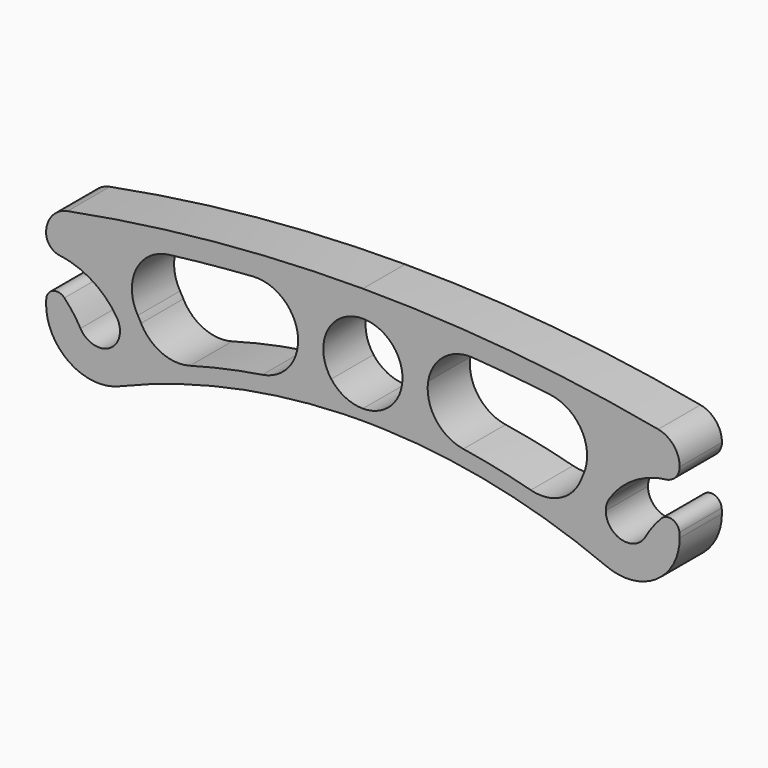
from build123d import *
from build123d import SkipClean  # not in build123d's __all__

# Parameters (mm, degrees)
F1_DEPTH    = 10
F3_R        = 5
F4_R        = 3
F5_R        = 2
F7_DEPTH    = 10.0010001
F8_T1_DEPTH = 10


# Not quite as in the source:
# - a fillet or chamfer that OpenCascade refuses, or shapes differently, is made with other operations: its cross-section is extruded or revolved along the edge and cut away or added


with BuildPart() as f1:
    # F0 (on Front) → F1 (new body)
    with BuildSketch(Plane.XZ):
        with BuildLine():
            ThreePointArc((-60, 9), (-57.6213157363, 8.9328971517), (-55.2831757887, 8.4904683961))
            ThreePointArc((-55.2831757887, 8.4904683961), (-45.1436514688, 8.7416176388), (-40, 0))
            ThreePointArc((-40, 0), (-41.6794970566, -5.5470019623), (-46.1538461538, -9.2307692308))
            ThreePointArc((-46.1538461538, -9.2307692308), (-25.4921003461, -2.7389543798), (-4, -0.0666851955))
            ThreePointArc((-4, -0.0666851955), (-4.6347028183, 2.6231856146), (-5.9814434357, 5.03659448))
            ThreePointArc((-5.9814434357, 5.03659448), (-6.715086481, 12.9015322824), (0, 17.061230866))
            Line((0, 17.061230866), (0, 22.061230866))
            ThreePointArc((0, 22.061230866), (-30.1526886016, 20.5420767676), (-60, 16))
            Line((-60, 16), (-60, 9))
        make_face()
        with BuildLine():
            ThreePointArc((-46.6427971379, 2.1746698468), (-46.1640639051, 1.1338404984), (-46, 0))
            ThreePointArc((-46, 0), (-48.9877288652, -3.8697941999), (-53.4876535749, -1.958640483))
            ThreePointArc((-53.4876535749, -1.958640483), (-55.921777017, 1.4722128283), (-59.0196729824, 4.3180434563))
            ThreePointArc((-59.0196729824, 4.3180434563), (-59.7518390528, 2.21396366), (-60, 0))
            ThreePointArc((-60, 0), (-55.5470019623, -8.3205029434), (-46.1538461538, -9.2307692308))
            ThreePointArc((-46.1538461538, -9.2307692308), (-41.6794970566, -5.5470019623), (-40, 0))
            ThreePointArc((-40, 0), (-45.1436514688, 8.7416176388), (-55.2831757887, 8.4904683961))
            ThreePointArc((-55.2831757887, 8.4904683961), (-50.3805281419, 6.1294058803), (-46.6427971379, 2.1746698468))
        make_face()
        with BuildLine():
            ThreePointArc((-5.9814434357, 5.03659448), (-4.6347028183, 2.6231856146), (-4, -0.0666851955))
            ThreePointArc((-4, -0.0666851955), (-2.0002779129, -0.0166724571), (0, 0))
            Line((0, 0), (0, 2.061230866))
            ThreePointArc((0, 2.061230866), (-3.3403014164, 2.846144385), (-5.9814434357, 5.03659448))
        make_face()
    extrude(amount=F1_DEPTH)

    # F2: F1 across plane


with BuildPart() as f1_1:
    add(f1.part, clean=False)
    with SkipClean():  # cleaning this boolean's faces spoils the solid; the shape is the same uncleaned
        add(f1.part.mirror(Plane.YZ), clean=False)

    # F3
    f3_edges = [f1_1.edges().sort_by_distance(p)[0] for p in [
        (-60, -5, 16),
        (60, -5, 16),
    ]]
    fillet(f3_edges, radius=F3_R)

    # F4
    f4_edges = [f1_1.edges().sort_by_distance(p)[0] for p in [
        (-60, -5, 9),
        (60, -5, 9),
    ]]
    fillet(f4_edges, radius=F4_R)

    # F5
    f5_edges = [f1_1.edges().sort_by_distance(p)[0] for p in [
        (-59.019673, -5, 4.318043),
        (59.019673, -5, 4.318043),
    ]]
    fillet(f5_edges, radius=F5_R)

    # F6 (on face) → F7 (cut, through all)
    with BuildSketch(Plane.XZ.offset(10)):
        with BuildLine():
            ThreePointArc((-7.8234196702, 2.7509433962), (-12.1811976175, 9.6949287705), (-11.2993718648, 17.8454836508))
            ThreePointArc((-11.2993718648, 17.8454836508), (-33.2415394106, 16.1887543276), (-55, 12.9065505808))
            ThreePointArc((-55, 12.9065505808), (-44.9636385736, 6.903343626), (-40, -3.685770432))
            ThreePointArc((-40, -3.685770432), (-24.1273224471, 0.6104154355), (-7.8234196702, 2.7509433962))
        make_face()
        with BuildLine():
            ThreePointArc((40, -3.685770432), (42.6359894717, 6.412330531), (50, 13.8076961402))
            ThreePointArc((50, 13.8076961402), (30.7161061945, 16.4632023612), (11.2993718648, 17.8454836508))
            ThreePointArc((11.2993718648, 17.8454836508), (12.1961499726, 15.2393294517), (12.5, 12.5))
            ThreePointArc((12.5, 12.5), (11.2703759005, 7.0936493768), (7.8234196702, 2.7509433962))
            ThreePointArc((7.8234196702, 2.7509433962), (24.1273224471, 0.6104154355), (40, -3.685770432))
        make_face()
    extrude(amount=-F7_DEPTH, mode=Mode.SUBTRACT)

    # F8: fillet of radius 8 on 8 edges, made by hand

    # F8_s2 → F8_t1 (join)
    with BuildSketch(Plane.XZ):
        with BuildLine():
            ThreePointArc((-36.7451179027, 15.7716261712), (-42.9406323526, 11.3440144515), (-42.6227863201, 3.7356559729))
            ThreePointArc((-42.6227863201, 3.7356559729), (-47.8930149535, 9.5605639606), (-55, 12.9065505808))
            ThreePointArc((-55, 12.9065505808), (-45.8949216066, 14.4815724477), (-36.7451179027, 15.7716261712))
        make_face()
        with BuildLine():
            ThreePointArc((-42.0039790926, 2.6185161763), (-38.1014001727, -1.0557269801), (-32.7552534978, -1.4416035521))
            ThreePointArc((-32.7552534978, -1.4416035521), (-36.3949282061, -2.5078334489), (-40, -3.685770432))
            ThreePointArc((-40, -3.685770432), (-40.7395345489, -0.4501990795), (-42.0039790926, 2.6185161763))
        make_face()
        with BuildLine():
            ThreePointArc((-12.3583566886, 10.623561896), (-13.8147498473, 4.6940719377), (-19.0299825284, 1.5189687455))
            ThreePointArc((-19.0299825284, 1.5189687455), (-13.4408237395, 2.2634215831), (-7.8234196702, 2.7509433962))
            ThreePointArc((-7.8234196702, 2.7509433962), (-10.83146134, 6.2606534605), (-12.3583566886, 10.623561896))
        make_face()
        with BuildLine():
            ThreePointArc((-12.3513599638, 10.578046035), (-15.2694424, 15.6035487131), (-20.8189034057, 17.3281834039))
            ThreePointArc((-20.8189034057, 17.3281834039), (-16.0612204229, 17.6251616805), (-11.2993718648, 17.8454836508))
            ThreePointArc((-11.2993718648, 17.8454836508), (-12.3710626618, 14.2907564373), (-12.3513599638, 10.578046035))
        make_face()
        with BuildLine():
            ThreePointArc((20.8189034057, 17.3281834039), (15.2694424, 15.6035487131), (12.3513599638, 10.578046035))
            ThreePointArc((12.3513599638, 10.578046035), (12.3710626618, 14.2907564373), (11.2993718648, 17.8454836508))
            ThreePointArc((11.2993718648, 17.8454836508), (16.0612204229, 17.6251616805), (20.8189034057, 17.3281834039))
        make_face()
        with BuildLine():
            ThreePointArc((12.3583566886, 10.623561896), (13.8147498473, 4.6940719377), (19.0299825284, 1.5189687455))
            ThreePointArc((19.0299825284, 1.5189687455), (13.4408237395, 2.2634215831), (7.8234196702, 2.7509433962))
            ThreePointArc((7.8234196702, 2.7509433962), (10.83146134, 6.2606534605), (12.3583566886, 10.623561896))
        make_face()
        with BuildLine():
            ThreePointArc((41.7652662923, 4.7039127832), (41.4390880083, 11.9220711187), (35.429216879, 15.9332618444))
            ThreePointArc((35.429216879, 15.9332618444), (42.7278279524, 14.9610989412), (50, 13.8076961402))
            ThreePointArc((50, 13.8076961402), (45.1669008636, 9.9032127448), (41.7652662923, 4.7039127832))
        make_face()
        with BuildLine():
            ThreePointArc((41.3345230553, 3.6720037672), (37.4981716447, -0.5831636355), (31.800316666, -1.1819043245))
            ThreePointArc((31.800316666, -1.1819043245), (35.9219808015, -2.3623729613), (40, -3.685770432))
            ThreePointArc((40, -3.685770432), (40.3203276581, 0.056042117), (41.3345230553, 3.6720037672))
        make_face()
    extrude(amount=F8_T1_DEPTH)


solid = f1_1.part
